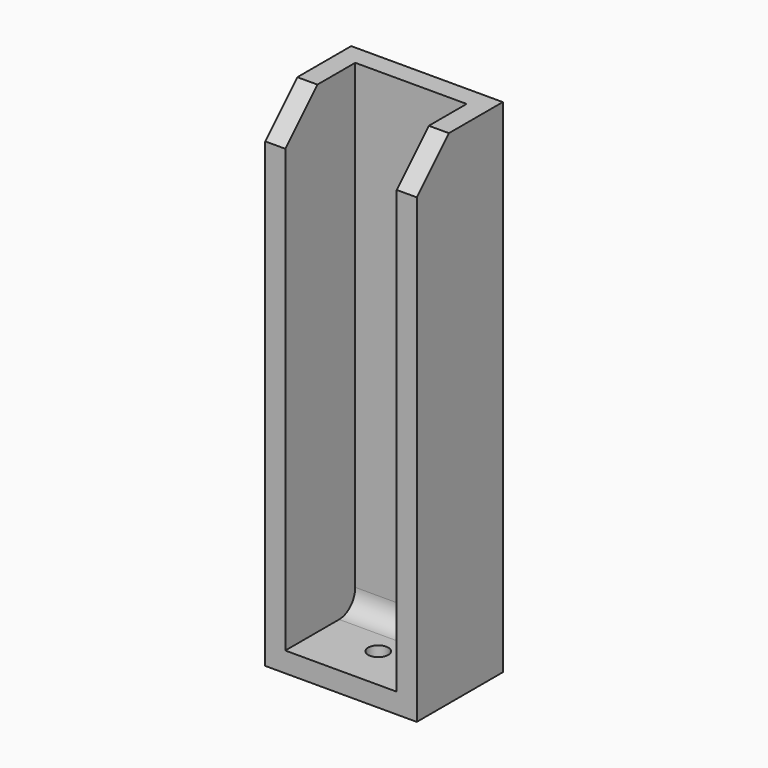
from build123d import *

# Parameters (mm, degrees)
F0_W        = 191.7510181665
F0_H        = 135.9910964966
F1_DEPTH    = 635
F2_T        = -25.4
F4_D        = 25.4
F5_R        = 25.4
F6_T1_DEPTH = 286.6829915773
F6_T3_DEPTH = 286.6829915773


# Not quite as in the source:
# - a fillet or chamfer that OpenCascade refuses, or shapes differently, is made with other operations: its cross-section is extruded or revolved along the edge and cut away or added


with BuildPart() as f1:
    # F0 (on Top) → F1 (new body)
    with BuildSketch(Plane.XY):
        with Locations((95.8755090833, 67.9955482483)):
            Rectangle(F0_W, F0_H)
    extrude(amount=F1_DEPTH)

    # F2
    f2_openings = [f1.faces().sort_by_distance(p)[0] for p in [
        (95.875509, 0, 317.5),
        (95.875509, 67.995548, 635),
    ]]
    offset(amount=F2_T, openings=f2_openings)

    # F4 (through all)
    with Locations(Plane.XY.offset(25.4)):
        with Locations((98.0245098472, 56.1208538711)):
            Hole(F4_D / 2)

    # F5
    f5_edges = [f1.edges().sort_by_distance(p)[0] for p in [
        (95.875509, 110.591096, 25.4),
    ]]
    fillet(f5_edges, radius=F5_R)

    # F6: chamfer of 50.8 on 3 edges, made by hand

    # F6_s2 → F6_t1 (cut)
    with BuildSketch(Plane.YZ.offset(-130.6414957887)):
        Polygon((0, 584.2), (50.8, 635), (0, 635), align=None)
    extrude(amount=F6_T1_DEPTH, mode=Mode.SUBTRACT)

    # F6_s4 → F6_t3 (cut)
    with BuildSketch(Plane.YZ.offset(35.7095223779)):
        Polygon((0, 584.2), (50.8, 635), (0, 635), align=None)
    extrude(amount=F6_T3_DEPTH, mode=Mode.SUBTRACT)


solid = f1.part
